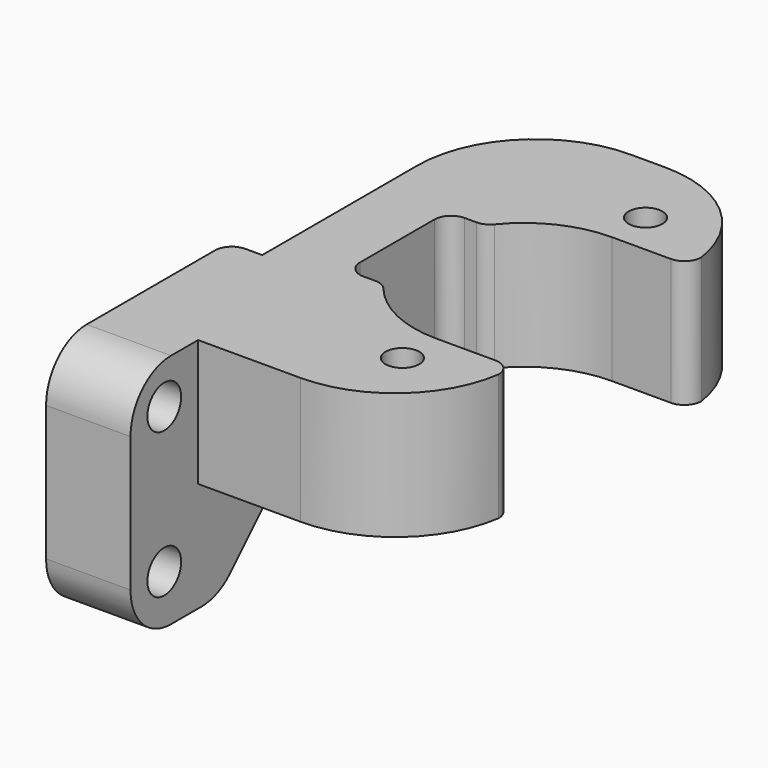
from build123d import *

# Parameters (mm, degrees)
F0_W          = 18
F0_H          = 32
F1_DEPTH      = 14
F2_W          = 13
F2_H          = 5
F2_W_2        = 2
F2_H_2        = 18.5
F3_DEPTH      = 14
F4_W          = 27
F4_H          = 6.5
F5_DEPTH      = 18.001
F6_R          = 1
F7_DEPTH      = 7.5
F8_R          = 1.25
F9_DEPTH      = 5
F10_T4_DEPTH  = 5
F11_T4_DEPTH  = 8.1066017178
F11_T9_DEPTH  = 8.1066017178
F11_T12_DEPTH = 20
F11_T14_DEPTH = 11.2132034356
F12_R         = 1
F13_T1_DEPTH  = 42.1410161514
F13_T3_DEPTH  = 42.5
F15_DEPTH     = 14.001
F16_R         = 1


# Not quite as in the source:
# - a fillet or chamfer that OpenCascade refuses, or shapes differently, is made with other operations: its cross-section is extruded or revolved along the edge and cut away or added


with BuildPart() as f1:
    # F0 (on Top) → F1 (new body)
    with BuildSketch(Plane.XY):
        with Locations((9, 16)):
            Rectangle(F0_W, F0_H)
    extrude(amount=F1_DEPTH)

    # F2 (on face) → F3 (cut, through all)
    with BuildSketch(Plane.XY.offset(14)):
        with Locations((11.5, 2.5)):
            Rectangle(F2_W, F2_H)
        with Locations((1, 22.75)):
            Rectangle(F2_W_2, F2_H_2)
    extrude(amount=-F3_DEPTH, mode=Mode.SUBTRACT)

    # F4 (on face) → F5 (cut, through all)
    with BuildSketch(Plane.YZ.offset(18)):
        with Locations((18.5, 3.25)):
            Rectangle(F4_W, F4_H)
    extrude(amount=-F5_DEPTH, mode=Mode.SUBTRACT)

    # F6 (on face) → F7 (cut, through all)
    with BuildSketch(Plane.XY.offset(14)):
        with Locations((13.5, 9.5)):
            Circle(F6_R)
        with BuildLine():
            ThreePointArc((18, 23.1904157598), (15.9251079936, 24.5306592691), (13.5, 25))
            ThreePointArc((13.5, 25), (7, 18.5), (13.5, 12))
            ThreePointArc((13.5, 12), (15.9251079936, 12.4693407309), (18, 13.8095842402))
            Line((18, 13.8095842402), (18, 23.1904157598))
        make_face()
        with Locations((13.5, 27.5)):
            Circle(F6_R)
        with BuildLine():
            Line((18, 25), (13.5, 25))
            ThreePointArc((13.5, 25), (15.9251079936, 24.5306592691), (18, 23.1904157598))
            Line((18, 23.1904157598), (18, 25))
        make_face()
        with BuildLine():
            ThreePointArc((18, 13.8095842402), (15.9251079936, 12.4693407309), (13.5, 12))
            Line((13.5, 12), (18, 12))
            Line((18, 12), (18, 13.8095842402))
        make_face()
    extrude(amount=-F7_DEPTH, mode=Mode.SUBTRACT)

    # F8 (on face) → F9 (cut, through all)
    with BuildSketch(Plane.YZ.offset(5)):
        with Locations((2.5, 11.55)):
            Circle(F8_R)
        with Locations((2.5, 2.95)):
            Circle(F8_R)
    extrude(amount=-F9_DEPTH, mode=Mode.SUBTRACT)

    # F10: chamfer of 8 on 1 edges, made by hand


with BuildPart() as f10_tool2:
    # F10_s3 → F10_t4 (new body)
    with BuildSketch(Plane.YZ.offset(5)):
        Polygon((5, -1.5), (13, 6.5), (5, 6.5), align=None)
    extrude(amount=-F10_T4_DEPTH)

    split(bisect_by=Plane.XY, keep=Keep.TOP)


with BuildPart() as f1_1:
    add(f1.part)

    # F10_t1: union F10_tool2
    add(f10_tool2.part)

    # F11: fillet of radius 3 on 5 edges, made by hand


with BuildPart() as f11_tool2:
    # F11_s3 → F11_t4 (new body)
    with BuildSketch(Plane.YZ.offset(5)):
        with BuildLine():
            ThreePointArc((14.2426406871, 6.5), (13.09459039, 6.2716385975), (12.1213203436, 5.6213203436))
            Line((12.1213203436, 5.6213203436), (13, 6.5))
            Line((13, 6.5), (14.2426406871, 6.5))
        make_face()
    extrude(amount=-F11_T4_DEPTH)

    split(bisect_by=Plane.YZ.offset(2), keep=Keep.TOP)


with BuildPart() as f1_2:
    add(f1_1.part)

    # F11_t1: union F11_tool2
    add(f11_tool2.part)


with BuildPart() as f11_tool7:
    # F11_s8 → F11_t9 (new body)
    with BuildSketch(Plane.YZ.offset(8.1066017178)):
        with BuildLine():
            ThreePointArc((14.2426406871, 6.5), (13.09459039, 6.2716385975), (12.1213203436, 5.6213203436))
            Line((12.1213203436, 5.6213203436), (13, 6.5))
            Line((13, 6.5), (14.2426406871, 6.5))
        make_face()
    extrude(amount=-F11_T9_DEPTH)

    split(bisect_by=Plane.YZ.offset(2), keep=Keep.BOTTOM)

    split(bisect_by=Plane.XZ.offset(-13.5), keep=Keep.TOP)


with BuildPart() as f1_3:
    add(f1_2.part)

    # F11_t6: union F11_tool7
    add(f11_tool7.part)

    # F11_s13 → F11_t12 (cut)
    with BuildSketch(Plane.YZ.offset(-7.5)):
        with BuildLine():
            ThreePointArc((0, 11), (0.8786796564, 13.1213203436), (3, 14))
            Line((3, 14), (0, 14))
            Line((0, 14), (0, 11))
        make_face()
        with BuildLine():
            ThreePointArc((0, 3), (0.8786796564, 0.8786796564), (3, 0))
            Line((3, 0), (0, 0))
            Line((0, 0), (0, 3))
        make_face()
    extrude(amount=F11_T12_DEPTH, mode=Mode.SUBTRACT)

    # F11_s15 → F11_t14 (cut)
    with BuildSketch(Plane.YZ.offset(-3.1066017178)):
        with BuildLine():
            ThreePointArc((7.3786796564, 0.8786796564), (6.40540961, 0.2283614025), (5.2573593129, 0))
            Line((5.2573593129, 0), (6.5, 0))
            Line((6.5, 0), (7.3786796564, 0.8786796564))
        make_face()
    extrude(amount=F11_T14_DEPTH, mode=Mode.SUBTRACT)

    # F12
    f12_edges = [f1_3.edges().sort_by_distance(p)[0] for p in [
        (18, 12, 10.25),
        (18, 25, 10.25),
    ]]
    fillet(f12_edges, radius=F12_R)

    # F13: fillet of radius 7 on 3 edges, made by hand

    # F13_s2 → F13_t1 (cut)
    with BuildSketch(Plane.XY.offset(-10.8205080757)):
        with BuildLine():
            ThreePointArc((18, 11), (15.6543724647, 6.7084973779), (11.0717967697, 5))
            Line((11.0717967697, 5), (11.0717967697, 4.86))
            Line((11.0717967697, 4.86), (18, 4.86))
            Line((18, 4.86), (18.14, 5))
            ThreePointArc((18.14, 5), (18.14, 8), (18.1385640646, 10.98))
            Line((18.1385640646, 10.98), (18, 11))
        make_face()
        with BuildLine():
            ThreePointArc((18, 26), (15.6543724647, 30.2915026221), (11.0717967697, 32))
            Line((11.0717967697, 32), (11.0717967697, 32.14))
            Line((11.0717967697, 32.14), (18, 32.14))
            Line((18, 32.14), (18.14, 32))
            ThreePointArc((18.14, 32), (18.14, 29), (18.1385640646, 26.02))
            Line((18.1385640646, 26.02), (18, 26))
        make_face()
    extrude(amount=F13_T1_DEPTH, mode=Mode.SUBTRACT)

    # F13_s4 → F13_t3 (cut)
    with BuildSketch(Plane.XY.offset(-11)):
        with BuildLine():
            ThreePointArc((9, 32), (4.0502525317, 29.9497474683), (2, 25))
            Line((2, 25), (1.86, 25))
            Line((1.86, 25), (1.86, 32.14))
            Line((1.86, 32.14), (9, 32.14))
            Line((9, 32.14), (9, 32))
        make_face()
    extrude(amount=F13_T3_DEPTH, mode=Mode.SUBTRACT)

    # F14 (on face) → F15 (cut, through all)
    with BuildSketch(Plane.XY.offset(14)):
        with BuildLine():
            ThreePointArc((8.1908098546, 14.75), (7, 18.5), (8.1908098546, 22.25))
            Line((8.1908098546, 22.25), (5.9908098546, 22.25))
            Line((5.9908098546, 22.25), (5.9908098546, 14.75))
            Line((5.9908098546, 14.75), (8.1908098546, 14.75))
        make_face()
    extrude(amount=-F15_DEPTH, mode=Mode.SUBTRACT)

    # F16
    f16_edges = [f1_3.edges().sort_by_distance(p)[0] for p in [
        (5.99081, 14.75, 10.25),
        (5.99081, 22.25, 10.25),
        (8.19081, 22.25, 10.25),
        (8.19081, 14.75, 10.25),
        (0, 13.5, 10.203314),
    ]]
    fillet(f16_edges, radius=F16_R)


solid = f1_3.part
